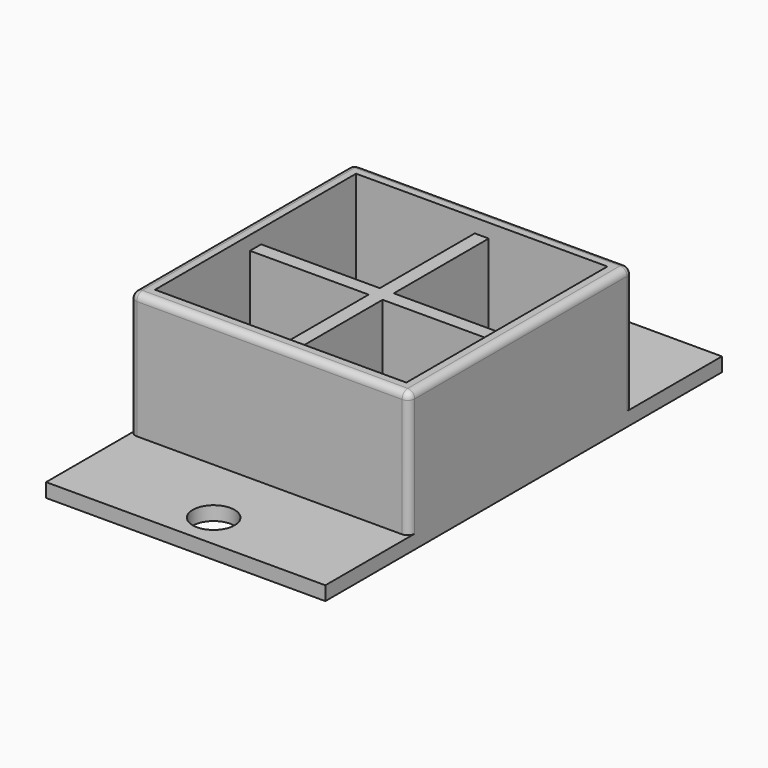
from build123d import *

# Parameters (mm, degrees)
F0_W     = 20
F0_H     = 20
F1_DEPTH = 10
F2_T     = -1
F4_DEPTH = 9
F5_W     = 20
F5_H     = 8
F5_R     = 1.5
F6_DEPTH = 1
F7_W     = 18
F7_H     = 18
F8_DEPTH = 1
F9_R     = 0.5


with BuildPart() as f1:
    # F0 (on Top) → F1 (new body)
    with BuildSketch(Plane.XY):
        Rectangle(F0_W, F0_H)
    extrude(amount=F1_DEPTH)

    # F2
    f2_openings = [f1.faces().sort_by_distance(p)[0] for p in [
        (0, 0, 0),
    ]]
    offset(amount=F2_T, openings=f2_openings)

    # F3 (on Top) → F4 (join)
    with BuildSketch(Plane.XY):
        Polygon((-0.5, -9), (0.5, -9), (0.5, -0.5), (9, -0.5), (9, 0.5), (0.5, 0.5), (0.5, 9), (-0.5, 9), (-0.5, 0.5), (-9, 0.5), (-9, -0.5), (-0.5, -0.5), align=None)
    extrude(amount=F4_DEPTH)

    # F5 (on Top) → F6 (join)
    with BuildSketch(Plane.XY):
        with Locations((0, -13.5)):
            Rectangle(F5_W, F5_H)
        with Locations((0, -15)):
            Circle(F5_R, mode=Mode.SUBTRACT)
        with Locations((0, 14)):
            Rectangle(F5_W, F5_H)
        with Locations((0, 15)):
            Circle(F5_R, mode=Mode.SUBTRACT)
    extrude(amount=F6_DEPTH)

    # F7 (on face) → F8 (cut)
    with BuildSketch(Plane.XY.offset(10)):
        Rectangle(F7_W, F7_H)
    extrude(amount=-F8_DEPTH, mode=Mode.SUBTRACT)

    # F9
    f9_edges = [f1.edges().sort_by_distance(p)[0] for p in [
        (0, -10, 10),
        (10, 0, 10),
        (10, -10, 5.5),
        (-10, -10, 5.5),
        (-10, 0, 10),
        (0, 10, 10),
        (10, 10, 5.5),
        (-10, 10, 5.5),
    ]]
    fillet(f9_edges, radius=F9_R)


solid = f1.part
